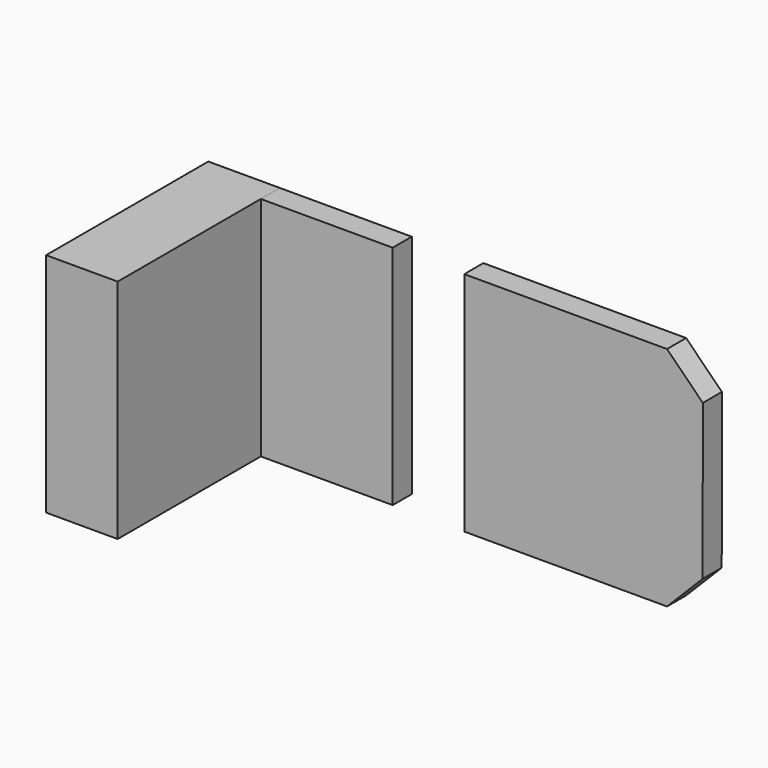
from build123d import *

# Parameters (mm, degrees)
F1_DEPTH = 12.7
F0_W     = 38.1
F0_H     = 120.65
F2_DEPTH = 107.95


# Not quite as in the source:
# - a feature names something its author has since deleted; it is built from what else it names


with BuildPart() as f1:
    # F0 (on Front) → F1 (new body)
    with BuildSketch(Plane.XZ):
        Polygon((-0.3467756933, 0), (0, 0), (69.85, 0), (69.85, 120.65), (-0.3467756933, 120.65), align=None)
    extrude(amount=F1_DEPTH)


with BuildPart() as f1b:
    # F0 (on Front) → F1, piece 2 (new body)
    with BuildSketch(Plane.XZ):
        Polygon((107.95, 120.65), (107.95, 0), (215.9, 0), (234.8521879996, 19.1473123447), (234.95, 101.6), (215.9, 120.65), align=None)
    extrude(amount=F1_DEPTH)


with BuildPart() as f2:
    # F0 (on Front) → F2 (new body)
    with BuildSketch(Plane.XZ):
        with Locations((-19.3967756933, 60.325)):
            Rectangle(F0_W, F0_H)
    extrude(amount=F2_DEPTH)


solid = Compound([f1.part, f1b.part, f2.part])
